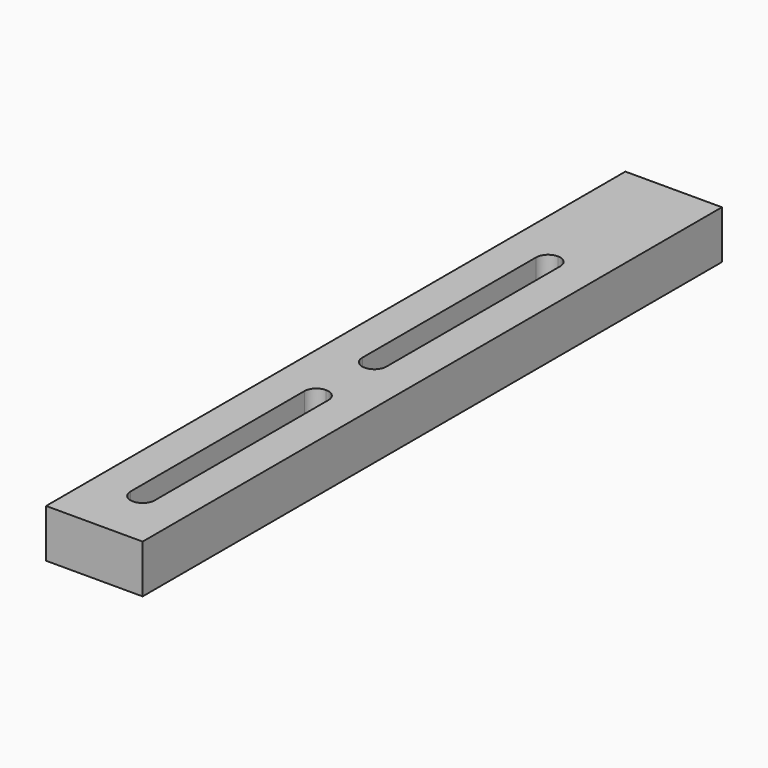
from build123d import *

# Parameters (mm, degrees)
F0_W     = 20
F0_H     = 150
F1_DEPTH = 10
F2_W     = 5
F2_H     = 50
F3_DEPTH = 25
F4_R     = 2.49999


# Not quite as in the source:
# - a fillet or chamfer is up to 0.001 mm smaller than in the source, because OpenCascade refuses the exact size


with BuildPart() as f1:
    # F0 (on Top) → F1 (new body)
    with BuildSketch(Plane.XY):
        with Locations((10, 75)):
            Rectangle(F0_W, F0_H)
    extrude(amount=F1_DEPTH)

    # F2 (on face) → F3 (cut)
    with BuildSketch(Plane.XY.offset(10)):
        with Locations((10, 95)):
            Rectangle(F2_W, F2_H)
        with Locations((10, 35)):
            Rectangle(F2_W, F2_H)
    extrude(amount=-F3_DEPTH, mode=Mode.SUBTRACT)

    # F4 (radius 2.5 in the source; OpenCascade refuses exactly that, so slightly less here)
    f4_edges = [f1.edges().sort_by_distance(p)[0] for p in [
        (12.5, 60, 5),
        (7.5, 60, 5),
        (7.5, 120, 5),
        (12.5, 120, 5),
        (7.5, 70, 5),
        (7.5, 10, 5),
        (12.5, 10, 5),
        (12.5, 70, 5),
    ]]
    fillet(f4_edges, radius=F4_R)


solid = f1.part
